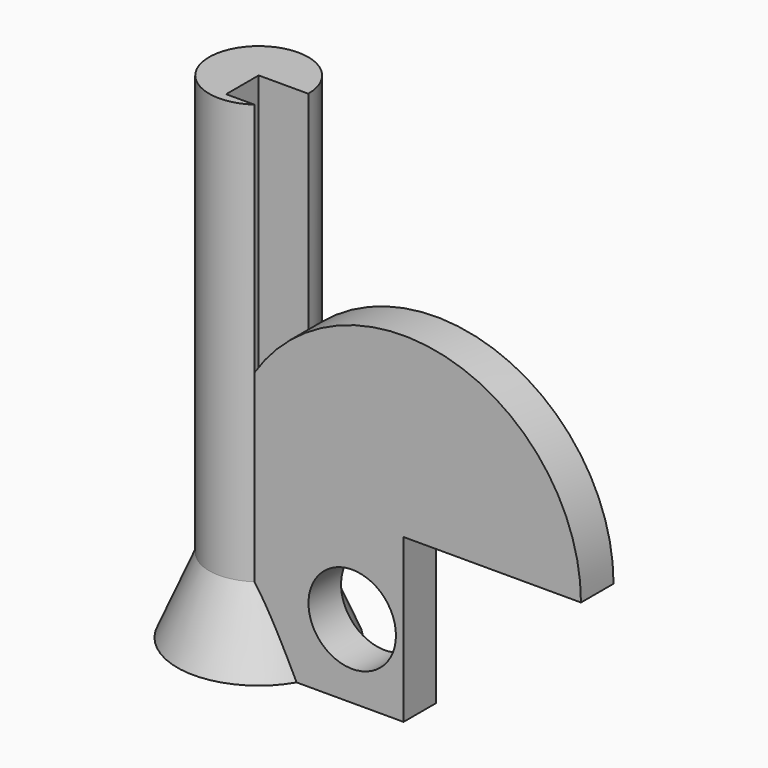
from build123d import *

# Parameters (mm, degrees)
F0_W     = 110.7262298465
F0_H     = 101.6
F0_R     = 27.2882199073
F1_DEPTH = 25.4
F4_DEPTH = 262.128
F5_ANGLE = 180


with BuildPart() as f1:
    # F0 (on Front) → F1 (new body)
    with BuildSketch(Plane.XZ):
        with Locations((55.3631149232, 50.8)):
            Rectangle(F0_W, F0_H)
        with Locations((78.689802438, 45.9539219737)):
            Circle(F0_R, mode=Mode.SUBTRACT)
    extrude(amount=F1_DEPTH)

    # F2 (on Front) → F3 (revolve)
    with BuildSketch(Plane.XZ):
        Polygon((-50.8, 0), (0, 0), (0, 46.7330427111), (-30.9378135865, 46.7330427111), align=None)
    revolve(axis=Axis((0, 0, 23.3665213556), (0, 0, -1)))

    # F4 (add): a face of the model
    f4_faces = [f1.faces().sort_by_distance(p)[0] for p in [
        (-4.0593514792, 3.4603008855, 46.7330427111),
    ]]
    extrude(f4_faces, amount=F4_DEPTH)

    # F1_face (on face) → F5 (revolve)
    with BuildSketch(Plane(origin=(55.3631149232, -12.7, 101.6), x_dir=(1, 0, 0), z_dir=(0, 0, 1))):
        Polygon((55.3631149232, -12.7), (55.3631149232, 12.7), (-24.4253013368, 12.7), (-55.3631149232, 12.7), (-55.3631149232, -12.7), (-37.6999241155, -12.7), align=None)
    revolve(axis=Axis((110.7262298465, -12.7, 101.6), (0, 1, 0)), revolution_arc=F5_ANGLE)


solid = f1.part
